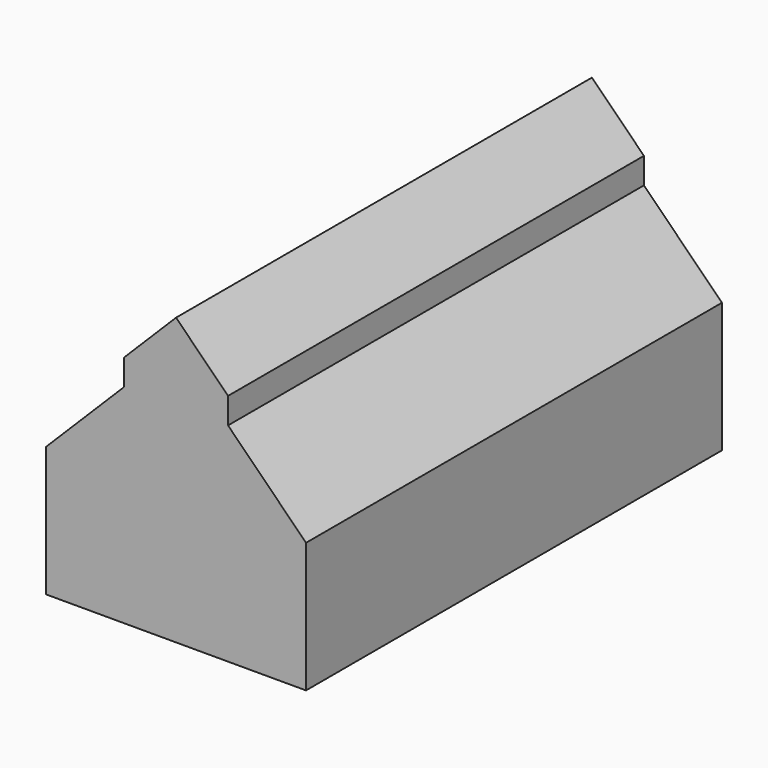
from build123d import *

# Parameters (mm, degrees)
F0_W     = 127
F0_H     = 101.6
F1_DEPTH = 254
F2_SIZE  = 38.1
F3_W     = 50.8
F3_H     = 254
F4_DEPTH = 38.1
F5_SIZE  = 25.39999


# Not quite as in the source:
# - a fillet or chamfer is up to 0.001 mm smaller than in the source, because OpenCascade refuses the exact size


with BuildPart() as f1:
    # F0 (on Front) → F1 (new body)
    with BuildSketch(Plane.XZ):
        with Locations((63.5, 50.8)):
            Rectangle(F0_W, F0_H)
    extrude(amount=F1_DEPTH)

    # F2
    f2_edges = [f1.edges().sort_by_distance(p)[0] for p in [
        (127, -127, 101.6),
        (0, -127, 101.6),
    ]]
    chamfer(f2_edges, length=F2_SIZE)

    # F3 (on face) → F4 (join)
    with BuildSketch(Plane.XY.offset(101.6)):
        with Locations((63.5, -127)):
            Rectangle(F3_W, F3_H)
    extrude(amount=F4_DEPTH)

    # F5 (size 25.4 in the source; OpenCascade refuses exactly that, so slightly less here)
    f5_edges = [f1.edges().sort_by_distance(p)[0] for p in [
        (38.1, -127, 139.7),
        (88.9, -127, 139.7),
    ]]
    chamfer(f5_edges, length=F5_SIZE)


solid = f1.part
